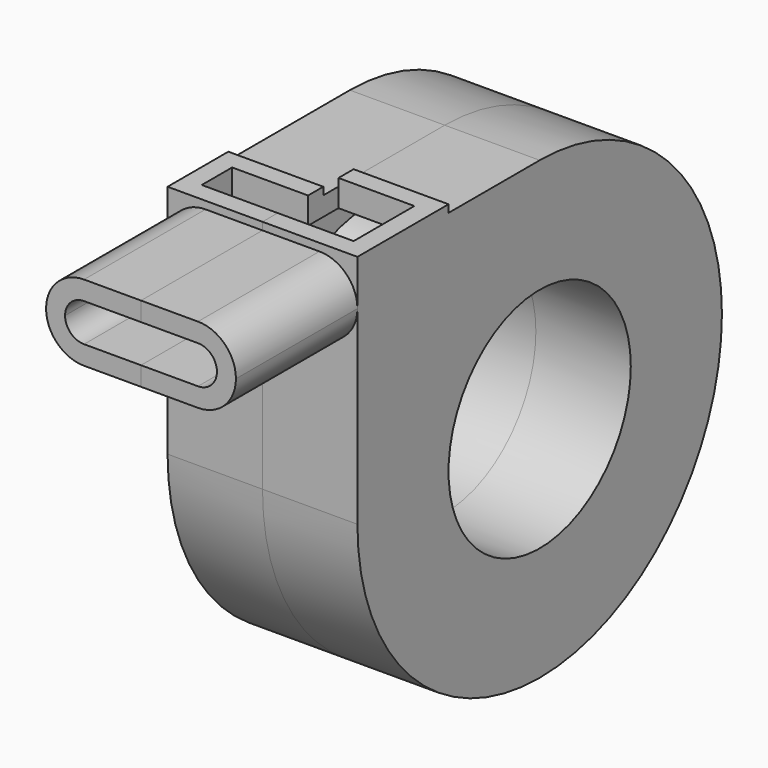
from build123d import *

# Parameters (mm, degrees)
F0_R     = 7.62
F0_W     = 5.08
F0_H     = 0.508
F1_DEPTH = 6.35
F2_T     = -1.27
F3_R     = 7.62
F3_W     = 7.62
F3_H     = 0.508
F4_DEPTH = 6.35
F5_T     = -1.27
F6_R     = 2.53999
F6_2_R   = 2.53999
F7_R     = 1.26999
F7_2_R   = 1.26999


# Not quite as in the source:
# - a fillet or chamfer is up to 0.001 mm smaller than in the source, because OpenCascade refuses the exact size


with BuildPart() as f1:
    # F0 (on Right) → F1 (new body)
    with BuildSketch(Plane.YZ):
        with BuildLine():
            Line((-15.24, 15.24), (-25.4, 15.24))
            Line((-25.4, 15.24), (-25.4, 10.16))
            Line((-25.4, 10.16), (-15.24, 10.16))
            Line((-15.24, 10.16), (-15.24, 0))
            ThreePointArc((-15.24, 0), (10.7763073453, -10.7763073453), (0, 15.24))
            Line((0, 15.24), (-10.16, 15.24))
            Line((-10.16, 15.24), (-15.24, 15.24))
        make_face()
        Circle(F0_R, mode=Mode.SUBTRACT)
        with Locations((-12.7, 15.494)):
            Rectangle(F0_W, F0_H)
    extrude(amount=-F1_DEPTH)

    # F2
    f2_openings = [f1.faces().sort_by_distance(p)[0] for p in [
        (-3.175, -25.4, 12.7),
        (-3.175, -12.7, 15.748),
        (0, -5.08, 14.728936),
    ]]
    offset(amount=F2_T, openings=f2_openings, kind=Kind.INTERSECTION)

    # F6 (radius 2.54 in the source; OpenCascade refuses exactly that, so slightly less here)
    f6_edges = [f1.edges().sort_by_distance(p)[0] for p in [
        (-6.35, -20.32, 15.24),
        (-6.35, -20.32, 10.16),
    ]]
    fillet(f6_edges, radius=F6_R)

    # F7 (radius 1.27 in the source; OpenCascade refuses exactly that, so slightly less here)
    f7_edges = [f1.edges().sort_by_distance(p)[0] for p in [
        (-5.08, -19.685, 13.97),
        (-5.08, -19.685, 11.43),
    ]]
    fillet(f7_edges, radius=F7_R)


with BuildPart() as f4:
    # F3 (on Right) → F4 (new body)
    with BuildSketch(Plane.YZ):
        with BuildLine():
            Line((-15.24, 15.24), (-25.4, 15.24))
            Line((-25.4, 15.24), (-25.4, 10.16))
            Line((-25.4, 10.16), (-15.24, 10.16))
            Line((-15.24, 10.16), (-15.24, 0))
            ThreePointArc((-15.24, 0), (10.7763073453, -10.7763073453), (0, 15.24))
            Line((0, 15.24), (-7.62, 15.24))
            Line((-7.62, 15.24), (-15.24, 15.24))
        make_face()
        Circle(F3_R, mode=Mode.SUBTRACT)
        with Locations((-11.43, 15.494)):
            Rectangle(F3_W, F3_H)
    extrude(amount=F4_DEPTH)

    # F5
    f5_openings = [f4.faces().sort_by_distance(p)[0] for p in [
        (3.175, -25.4, 12.7),
        (3.175, -11.43, 15.748),
        (0, -3.81, 14.728936),
    ]]
    offset(amount=F5_T, openings=f5_openings, kind=Kind.INTERSECTION)

    # F6#2 (radius 2.54 in the source; OpenCascade refuses exactly that, so slightly less here)
    f6_2_edges = [f4.edges().sort_by_distance(p)[0] for p in [
        (6.35, -20.32, 15.24),
        (6.35, -20.32, 10.16),
    ]]
    fillet(f6_2_edges, radius=F6_2_R)

    # F7#2 (radius 1.27 in the source; OpenCascade refuses exactly that, so slightly less here)
    f7_2_edges = [f4.edges().sort_by_distance(p)[0] for p in [
        (5.08, -19.685, 11.43),
        (5.08, -19.685, 13.97),
    ]]
    fillet(f7_2_edges, radius=F7_2_R)


solid = Compound([f1.part, f4.part])
